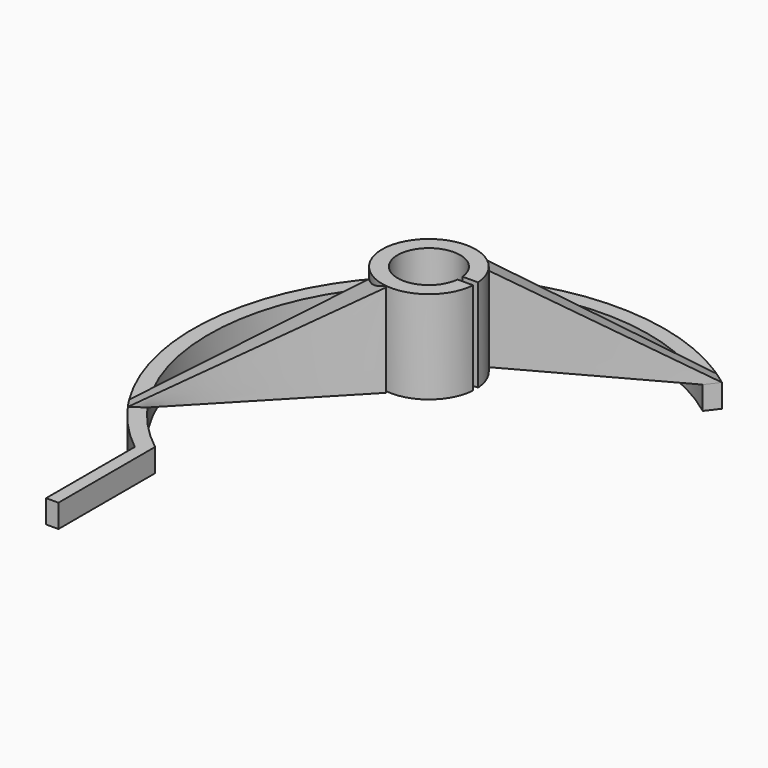
from build123d import *

# Parameters (mm, degrees)
F1_DEPTH = 3
F4_DEPTH = 12
F7_W     = 4
F7_H     = 12
F10_W    = 3
F10_H    = 12


# Not quite as in the source:
# - a feature of the source that left no trace in its solid (it failed there, or was rolled back) is left out
# - the arcs of a loft's sections are written as splines that run evenly, so that the points pair up as in the source's solid


with BuildPart() as f1:
    # F0 (on Top) → F1 (new body)
    with BuildSketch(Plane.XY):
        with BuildLine():
            ThreePointArc((-17.3497007267, 15.6394298017), (-22.6105701983, 55.5997007267), (17.3497007267, 60.8605701983))
            Line((17.3497007267, 60.8605701983), (18.5672235848, 62.4472768789))
            ThreePointArc((18.5672235848, 62.4472768789), (-24.0488636903, 57.0090552855), (-18.9497007267, 14.3510702673))
            ThreePointArc((-18.9497007267, 14.3510702673), (-18.1593804565, 13.7451657537), (-17.3497007267, 13.1653854984))
            Line((-17.3497007267, 13.1653854984), (-17.3497007267, 15.6394298017))
        make_face()
        with BuildLine():
            Line((-17.3497007267, 0), (-17.3497007267, 13.1653854984))
            ThreePointArc((-17.3497007267, 13.1653854984), (-18.1593804565, 13.7451657537), (-18.9497007267, 14.3510702673))
            Line((-18.9497007267, 14.3510702673), (-18.9497007267, 0))
            Line((-18.9497007267, 0), (-17.3497007267, 0))
        make_face()
    extrude(amount=F1_DEPTH)


with BuildPart() as f4:
    # F3 (on offset) → F4 (new body)
    with BuildSketch(Plane.XY.offset(8)):
        with BuildLine():
            ThreePointArc((4.0301985063, 37.85), (-4.05, 38.25), (4.0301985063, 38.65))
            Line((4.0301985063, 38.65), (6.0367623773, 38.65))
            ThreePointArc((6.0367623773, 38.65), (-6.05, 38.25), (6.0367623773, 37.85))
            Line((6.0367623773, 37.85), (4.0301985063, 37.85))
        make_face()
    extrude(amount=F4_DEPTH)


with BuildPart() as f8:
    # F7 (on face) → F8 section 0
    with BuildSketch(Plane(origin=(14.6540555932, 10.2608801917, 0), x_dir=(-0.5735764364, 0.8191520443, 0), z_dir=(0.8191520443, 0.5735764364, 0))):
        with Locations((28.4810658991, 14)):
            Rectangle(F7_W, F7_H)
    # F5 (on face) → F8 section 1
    with BuildSketch(Plane.XY.offset(3)):
        with BuildLine():
            Line((-24.22673654, 23.2394957905), (-25.8674584367, 22.0906499503))
            ThreePointArc((-25.8674584367, 22.0906499503), (-25.4345547517, 21.4174890589), (-24.9841373508, 20.7559186913))
            Line((-24.9841373508, 20.7559186913), (-23.3458332622, 21.903071564))
            ThreePointArc((-23.3458332622, 21.903071564), (-23.7956688669, 22.5650982415), (-24.22673654, 23.2394957905))
        make_face()
    loft()


with BuildPart() as f11:
    # F10 (on face) → F11 section 0
    with BuildSketch(Plane(origin=(20.9388152153, 27.2879952658, 0), x_dir=(-0.7933533403, 0.608761429, 0), z_dir=(0.608761429, 0.7933533403, 0))):
        with Locations((25.2521627247, 14)):
            Rectangle(F10_W, F10_H)
    # F5 (on face) → F11 section 1
    with BuildSketch(Plane.XY.offset(3)):
        with BuildLine():
            add(Edge.make_bspline(
                [(18.5672235848, 62.4472768789), (18.0379415831, 62.853409243), (17.4953295888, 63.2421692839), (16.9405551176, 63.6127205226)],
                knots=[0, 0, 0, 0, 1, 1, 1, 1], degree=3))
            Line((16.9405551176, 63.6127205226), (15.7202212212, 62.0223504256))
            add(Edge.make_bspline(
                [(15.7202212212, 62.0223504256), (16.276757018, 61.6543234662), (16.8203634304, 61.2667449915), (17.3497007267, 60.8605701983)],
                knots=[0, 0, 0, 0, 1, 1, 1, 1], degree=3))
            Line((17.3497007267, 60.8605701983), (18.5672235848, 62.4472768789))
        make_face()
    loft(ruled=True)


solid = Compound([f1.part, f4.part, f8.part, f11.part])
